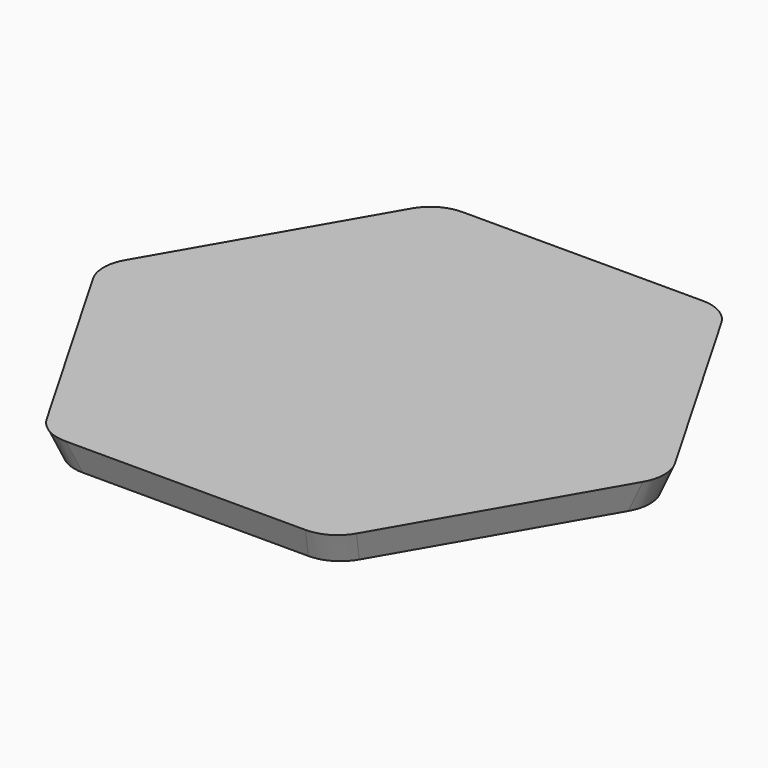
from build123d import *

# Parameters (mm, degrees)
F1_DEPTH = 5
F1_TAPER = -30
F3_DEPTH = 3
F3_TAPER = 30
F4_R     = 47.5
F5_DEPTH = 7
F5_TAPER = 22.5
F6_R     = 10


with BuildPart() as f1:
    # F0 (on Top) → F1 (new body)
    with BuildSketch(Plane.XY):
        Polygon((31.25, -54.1265877365), (62.5, 0), (31.25, 54.1265877365), (-31.25, 54.1265877365), (-62.5, 0), (-31.25, -54.1265877365), align=None)
    extrude(amount=F1_DEPTH, taper=F1_TAPER)

    # F2 (on face) → F3 (cut)
    with BuildSketch(Plane(origin=(0, 0, 0), x_dir=(1, 0, 0), z_dir=(0, 0, -1))):
        Polygon((61.1051684355, 65.1476408745), (58.6051684355, 60.8175138556), (61.1051684355, 56.4873868367), (66.1051684355, 56.4873868367), (68.6051684355, 60.8175138556), (66.1051684355, 65.1476408745), align=None)
        Polygon((51.440104926, 70.7277678934), (48.940104926, 66.3976408745), (51.440104926, 62.0675138556), (56.440104926, 62.0675138556), (58.940104926, 66.3976408745), (56.440104926, 70.7277678934), align=None)
        Polygon((48.940104926, 55.2376408745), (51.440104926, 50.9075138556), (56.440104926, 50.9075138556), (58.940104926, 55.2376408745), (56.440104926, 59.5677678934), (51.440104926, 59.5677678934), align=None)
        Polygon((66.1051684355, 53.9876408745), (61.1051684355, 53.9876408745), (58.6051684355, 49.6575138556), (61.1051684355, 45.3273868367), (66.1051684355, 45.3273868367), (68.6051684355, 49.6575138556), align=None)
        Polygon((48.940104926, 44.0776408745), (51.440104926, 39.7475138556), (56.440104926, 39.7475138556), (58.940104926, 44.0776408745), (56.440104926, 48.4077678934), (51.440104926, 48.4077678934), align=None)
        Polygon((66.1051684355, 42.8276408745), (61.1051684355, 42.8276408745), (58.6051684355, 38.4975138556), (61.1051684355, 34.1673868367), (66.1051684355, 34.1673868367), (68.6051684355, 38.4975138556), align=None)
        Polygon((48.940104926, 32.9176408745), (51.440104926, 28.5875138556), (56.440104926, 28.5875138556), (58.940104926, 32.9176408745), (56.440104926, 37.2477678934), (51.440104926, 37.2477678934), align=None)
        Polygon((66.1051684355, 31.6676408745), (61.1051684355, 31.6676408745), (58.6051684355, 27.3375138556), (61.1051684355, 23.0073868367), (66.1051684355, 23.0073868367), (68.6051684355, 27.3375138556), align=None)
        Polygon((48.940104926, 21.7576408745), (51.440104926, 17.4275138556), (56.440104926, 17.4275138556), (58.940104926, 21.7576408745), (56.440104926, 26.0877678934), (51.440104926, 26.0877678934), align=None)
        Polygon((66.1051684355, 20.5076408745), (61.1051684355, 20.5076408745), (58.6051684355, 16.1775138556), (61.1051684355, 11.8473868367), (66.1051684355, 11.8473868367), (68.6051684355, 16.1775138556), align=None)
        Polygon((48.940104926, 10.5976408745), (51.440104926, 6.2675138556), (56.440104926, 6.2675138556), (58.940104926, 10.5976408745), (56.440104926, 14.9277678934), (51.440104926, 14.9277678934), align=None)
        Polygon((66.1051684355, 9.3476408745), (61.1051684355, 9.3476408745), (58.6051684355, 5.0175138556), (61.1051684355, 0.6873868367), (66.1051684355, 0.6873868367), (68.6051684355, 5.0175138556), align=None)
        Polygon((48.940104926, -0.5623591255), (51.440104926, -4.8924861444), (56.440104926, -4.8924861444), (58.940104926, -0.5623591255), (56.440104926, 3.7677678934), (51.440104926, 3.7677678934), align=None)
        Polygon((66.1051684355, -1.8123591255), (61.1051684355, -1.8123591255), (58.6051684355, -6.1424861444), (61.1051684355, -10.4726131633), (66.1051684355, -10.4726131633), (68.6051684355, -6.1424861444), align=None)
        Polygon((48.940104926, -11.7223591255), (51.440104926, -16.0524861444), (56.440104926, -16.0524861444), (58.940104926, -11.7223591255), (56.440104926, -7.3922321066), (51.440104926, -7.3922321066), align=None)
        Polygon((66.1051684355, -12.9723591255), (61.1051684355, -12.9723591255), (58.6051684355, -17.3024861444), (61.1051684355, -21.6326131633), (66.1051684355, -21.6326131633), (68.6051684355, -17.3024861444), align=None)
        Polygon((48.940104926, -22.8823591255), (51.440104926, -27.2124861444), (56.440104926, -27.2124861444), (58.940104926, -22.8823591255), (56.440104926, -18.5522321066), (51.440104926, -18.5522321066), align=None)
        Polygon((66.1051684355, -24.1323591255), (61.1051684355, -24.1323591255), (58.6051684355, -28.4624861444), (61.1051684355, -32.7926131633), (66.1051684355, -32.7926131633), (68.6051684355, -28.4624861444), align=None)
        Polygon((48.940104926, -34.0423591255), (51.440104926, -38.3724861444), (56.440104926, -38.3724861444), (58.940104926, -34.0423591255), (56.440104926, -29.7122321066), (51.440104926, -29.7122321066), align=None)
        Polygon((66.1051684355, -35.2923591255), (61.1051684355, -35.2923591255), (58.6051684355, -39.6224861444), (61.1051684355, -43.9526131633), (66.1051684355, -43.9526131633), (68.6051684355, -39.6224861444), align=None)
        Polygon((48.940104926, -45.2023591255), (51.440104926, -49.5324861444), (56.440104926, -49.5324861444), (58.940104926, -45.2023591255), (56.440104926, -40.8722321066), (51.440104926, -40.8722321066), align=None)
        Polygon((66.1051684355, -46.4523591255), (61.1051684355, -46.4523591255), (58.6051684355, -50.7824861444), (61.1051684355, -55.1126131633), (66.1051684355, -55.1126131633), (68.6051684355, -50.7824861444), align=None)
        Polygon((28.940104926, 66.3976408745), (31.440104926, 62.0675138556), (36.440104926, 62.0675138556), (38.940104926, 66.3976408745), (36.440104926, 70.7277678934), (31.440104926, 70.7277678934), align=None)
        Polygon((46.1051684355, 65.1476408745), (41.1051684355, 65.1476408745), (38.6051684355, 60.8175138556), (41.1051684355, 56.4873868367), (46.1051684355, 56.4873868367), (48.6051684355, 60.8175138556), align=None)
        Polygon((28.940104926, 55.2376408745), (31.440104926, 50.9075138556), (36.440104926, 50.9075138556), (38.940104926, 55.2376408745), (36.440104926, 59.5677678934), (31.440104926, 59.5677678934), align=None)
        Polygon((46.1051684355, 53.9876408745), (41.1051684355, 53.9876408745), (38.6051684355, 49.6575138556), (41.1051684355, 45.3273868367), (46.1051684355, 45.3273868367), (48.6051684355, 49.6575138556), align=None)
        Polygon((28.940104926, 44.0776408745), (31.440104926, 39.7475138556), (36.440104926, 39.7475138556), (38.940104926, 44.0776408745), (36.440104926, 48.4077678934), (31.440104926, 48.4077678934), align=None)
        Polygon((46.1051684355, 42.8276408745), (41.1051684355, 42.8276408745), (38.6051684355, 38.4975138556), (41.1051684355, 34.1673868367), (46.1051684355, 34.1673868367), (48.6051684355, 38.4975138556), align=None)
        Polygon((28.940104926, 32.9176408745), (31.440104926, 28.5875138556), (36.440104926, 28.5875138556), (38.940104926, 32.9176408745), (36.440104926, 37.2477678934), (31.440104926, 37.2477678934), align=None)
        Polygon((46.1051684355, 31.6676408745), (41.1051684355, 31.6676408745), (38.6051684355, 27.3375138556), (41.1051684355, 23.0073868367), (46.1051684355, 23.0073868367), (48.6051684355, 27.3375138556), align=None)
        Polygon((28.940104926, 21.7576408745), (31.440104926, 17.4275138556), (36.440104926, 17.4275138556), (38.940104926, 21.7576408745), (36.440104926, 26.0877678934), (31.440104926, 26.0877678934), align=None)
        Polygon((46.1051684355, 20.5076408745), (41.1051684355, 20.5076408745), (38.6051684355, 16.1775138556), (41.1051684355, 11.8473868367), (46.1051684355, 11.8473868367), (48.6051684355, 16.1775138556), align=None)
        Polygon((28.940104926, 10.5976408745), (31.440104926, 6.2675138556), (36.440104926, 6.2675138556), (38.940104926, 10.5976408745), (36.440104926, 14.9277678934), (31.440104926, 14.9277678934), align=None)
        Polygon((46.1051684355, 9.3476408745), (41.1051684355, 9.3476408745), (38.6051684355, 5.0175138556), (41.1051684355, 0.6873868367), (46.1051684355, 0.6873868367), (48.6051684355, 5.0175138556), align=None)
        Polygon((28.940104926, -0.5623591255), (31.440104926, -4.8924861444), (36.440104926, -4.8924861444), (38.940104926, -0.5623591255), (36.440104926, 3.7677678934), (31.440104926, 3.7677678934), align=None)
        Polygon((46.1051684355, -1.8123591255), (41.1051684355, -1.8123591255), (38.6051684355, -6.1424861444), (41.1051684355, -10.4726131633), (46.1051684355, -10.4726131633), (48.6051684355, -6.1424861444), align=None)
        Polygon((28.940104926, -11.7223591255), (31.440104926, -16.0524861444), (36.440104926, -16.0524861444), (38.940104926, -11.7223591255), (36.440104926, -7.3922321066), (31.440104926, -7.3922321066), align=None)
        Polygon((46.1051684355, -12.9723591255), (41.1051684355, -12.9723591255), (38.6051684355, -17.3024861444), (41.1051684355, -21.6326131633), (46.1051684355, -21.6326131633), (48.6051684355, -17.3024861444), align=None)
        Polygon((28.940104926, -22.8823591255), (31.440104926, -27.2124861444), (36.440104926, -27.2124861444), (38.940104926, -22.8823591255), (36.440104926, -18.5522321066), (31.440104926, -18.5522321066), align=None)
        Polygon((46.1051684355, -24.1323591255), (41.1051684355, -24.1323591255), (38.6051684355, -28.4624861444), (41.1051684355, -32.7926131633), (46.1051684355, -32.7926131633), (48.6051684355, -28.4624861444), align=None)
        Polygon((28.940104926, -34.0423591255), (31.440104926, -38.3724861444), (36.440104926, -38.3724861444), (38.940104926, -34.0423591255), (36.440104926, -29.7122321066), (31.440104926, -29.7122321066), align=None)
        Polygon((46.1051684355, -35.2923591255), (41.1051684355, -35.2923591255), (38.6051684355, -39.6224861444), (41.1051684355, -43.9526131633), (46.1051684355, -43.9526131633), (48.6051684355, -39.6224861444), align=None)
        Polygon((28.940104926, -45.2023591255), (31.440104926, -49.5324861444), (36.440104926, -49.5324861444), (38.940104926, -45.2023591255), (36.440104926, -40.8722321066), (31.440104926, -40.8722321066), align=None)
        Polygon((46.1051684355, -46.4523591255), (41.1051684355, -46.4523591255), (38.6051684355, -50.7824861444), (41.1051684355, -55.1126131633), (46.1051684355, -55.1126131633), (48.6051684355, -50.7824861444), align=None)
        Polygon((8.940104926, 66.3976408745), (11.440104926, 62.0675138556), (16.440104926, 62.0675138556), (18.940104926, 66.3976408745), (16.440104926, 70.7277678934), (11.440104926, 70.7277678934), align=None)
        Polygon((26.1051684355, 65.1476408745), (21.1051684355, 65.1476408745), (18.6051684355, 60.8175138556), (21.1051684355, 56.4873868367), (26.1051684355, 56.4873868367), (28.6051684355, 60.8175138556), align=None)
        Polygon((8.940104926, 55.2376408745), (11.440104926, 50.9075138556), (16.440104926, 50.9075138556), (18.940104926, 55.2376408745), (16.440104926, 59.5677678934), (11.440104926, 59.5677678934), align=None)
        Polygon((26.1051684355, 53.9876408745), (21.1051684355, 53.9876408745), (18.6051684355, 49.6575138556), (21.1051684355, 45.3273868367), (26.1051684355, 45.3273868367), (28.6051684355, 49.6575138556), align=None)
        Polygon((8.940104926, 44.0776408745), (11.440104926, 39.7475138556), (16.440104926, 39.7475138556), (18.940104926, 44.0776408745), (16.440104926, 48.4077678934), (11.440104926, 48.4077678934), align=None)
        Polygon((26.1051684355, 42.8276408745), (21.1051684355, 42.8276408745), (18.6051684355, 38.4975138556), (21.1051684355, 34.1673868367), (26.1051684355, 34.1673868367), (28.6051684355, 38.4975138556), align=None)
        Polygon((8.940104926, 32.9176408745), (11.440104926, 28.5875138556), (16.440104926, 28.5875138556), (18.940104926, 32.9176408745), (16.440104926, 37.2477678934), (11.440104926, 37.2477678934), align=None)
        Polygon((26.1051684355, 31.6676408745), (21.1051684355, 31.6676408745), (18.6051684355, 27.3375138556), (21.1051684355, 23.0073868367), (26.1051684355, 23.0073868367), (28.6051684355, 27.3375138556), align=None)
        Polygon((8.940104926, 21.7576408745), (11.440104926, 17.4275138556), (16.440104926, 17.4275138556), (18.940104926, 21.7576408745), (16.440104926, 26.0877678934), (11.440104926, 26.0877678934), align=None)
        Polygon((26.1051684355, 20.5076408745), (21.1051684355, 20.5076408745), (18.6051684355, 16.1775138556), (21.1051684355, 11.8473868367), (26.1051684355, 11.8473868367), (28.6051684355, 16.1775138556), align=None)
        Polygon((8.940104926, 10.5976408745), (11.440104926, 6.2675138556), (16.440104926, 6.2675138556), (18.940104926, 10.5976408745), (16.440104926, 14.9277678934), (11.440104926, 14.9277678934), align=None)
        Polygon((26.1051684355, 9.3476408745), (21.1051684355, 9.3476408745), (18.6051684355, 5.0175138556), (21.1051684355, 0.6873868367), (26.1051684355, 0.6873868367), (28.6051684355, 5.0175138556), align=None)
        Polygon((8.940104926, -0.5623591255), (11.440104926, -4.8924861444), (16.440104926, -4.8924861444), (18.940104926, -0.5623591255), (16.440104926, 3.7677678934), (11.440104926, 3.7677678934), align=None)
        Polygon((26.1051684355, -1.8123591255), (21.1051684355, -1.8123591255), (18.6051684355, -6.1424861444), (21.1051684355, -10.4726131633), (26.1051684355, -10.4726131633), (28.6051684355, -6.1424861444), align=None)
        Polygon((8.940104926, -11.7223591255), (11.440104926, -16.0524861444), (16.440104926, -16.0524861444), (18.940104926, -11.7223591255), (16.440104926, -7.3922321066), (11.440104926, -7.3922321066), align=None)
        Polygon((26.1051684355, -12.9723591255), (21.1051684355, -12.9723591255), (18.6051684355, -17.3024861444), (21.1051684355, -21.6326131633), (26.1051684355, -21.6326131633), (28.6051684355, -17.3024861444), align=None)
        Polygon((8.940104926, -22.8823591255), (11.440104926, -27.2124861444), (16.440104926, -27.2124861444), (18.940104926, -22.8823591255), (16.440104926, -18.5522321066), (11.440104926, -18.5522321066), align=None)
        Polygon((26.1051684355, -24.1323591255), (21.1051684355, -24.1323591255), (18.6051684355, -28.4624861444), (21.1051684355, -32.7926131633), (26.1051684355, -32.7926131633), (28.6051684355, -28.4624861444), align=None)
        Polygon((8.940104926, -34.0423591255), (11.440104926, -38.3724861444), (16.440104926, -38.3724861444), (18.940104926, -34.0423591255), (16.440104926, -29.7122321066), (11.440104926, -29.7122321066), align=None)
        Polygon((26.1051684355, -35.2923591255), (21.1051684355, -35.2923591255), (18.6051684355, -39.6224861444), (21.1051684355, -43.9526131633), (26.1051684355, -43.9526131633), (28.6051684355, -39.6224861444), align=None)
        Polygon((8.940104926, -45.2023591255), (11.440104926, -49.5324861444), (16.440104926, -49.5324861444), (18.940104926, -45.2023591255), (16.440104926, -40.8722321066), (11.440104926, -40.8722321066), align=None)
        Polygon((26.1051684355, -46.4523591255), (21.1051684355, -46.4523591255), (18.6051684355, -50.7824861444), (21.1051684355, -55.1126131633), (26.1051684355, -55.1126131633), (28.6051684355, -50.7824861444), align=None)
        Polygon((-11.059895074, 66.3976408745), (-8.559895074, 62.0675138556), (-3.559895074, 62.0675138556), (-1.059895074, 66.3976408745), (-3.559895074, 70.7277678934), (-8.559895074, 70.7277678934), align=None)
        Polygon((6.1051684355, 65.1476408745), (1.1051684355, 65.1476408745), (-1.3948315645, 60.8175138556), (1.1051684355, 56.4873868367), (6.1051684355, 56.4873868367), (8.6051684355, 60.8175138556), align=None)
        Polygon((-11.059895074, 55.2376408745), (-8.559895074, 50.9075138556), (-3.559895074, 50.9075138556), (-1.059895074, 55.2376408745), (-3.559895074, 59.5677678934), (-8.559895074, 59.5677678934), align=None)
        Polygon((6.1051684355, 53.9876408745), (1.1051684355, 53.9876408745), (-1.3948315645, 49.6575138556), (1.1051684355, 45.3273868367), (6.1051684355, 45.3273868367), (8.6051684355, 49.6575138556), align=None)
        Polygon((-11.059895074, 44.0776408745), (-8.559895074, 39.7475138556), (-3.559895074, 39.7475138556), (-1.059895074, 44.0776408745), (-3.559895074, 48.4077678934), (-8.559895074, 48.4077678934), align=None)
        Polygon((6.1051684355, 42.8276408745), (1.1051684355, 42.8276408745), (-1.3948315645, 38.4975138556), (1.1051684355, 34.1673868367), (6.1051684355, 34.1673868367), (8.6051684355, 38.4975138556), align=None)
        Polygon((-11.059895074, 32.9176408745), (-8.559895074, 28.5875138556), (-3.559895074, 28.5875138556), (-1.059895074, 32.9176408745), (-3.559895074, 37.2477678934), (-8.559895074, 37.2477678934), align=None)
        Polygon((6.1051684355, 31.6676408745), (1.1051684355, 31.6676408745), (-1.3948315645, 27.3375138556), (1.1051684355, 23.0073868367), (6.1051684355, 23.0073868367), (8.6051684355, 27.3375138556), align=None)
        Polygon((-11.059895074, 21.7576408745), (-8.559895074, 17.4275138556), (-3.559895074, 17.4275138556), (-1.059895074, 21.7576408745), (-3.559895074, 26.0877678934), (-8.559895074, 26.0877678934), align=None)
        Polygon((6.1051684355, 20.5076408745), (1.1051684355, 20.5076408745), (-1.3948315645, 16.1775138556), (1.1051684355, 11.8473868367), (6.1051684355, 11.8473868367), (8.6051684355, 16.1775138556), align=None)
        Polygon((-11.059895074, 10.5976408745), (-8.559895074, 6.2675138556), (-3.559895074, 6.2675138556), (-1.059895074, 10.5976408745), (-3.559895074, 14.9277678934), (-8.559895074, 14.9277678934), align=None)
        Polygon((6.1051684355, 9.3476408745), (1.1051684355, 9.3476408745), (-1.3948315645, 5.0175138556), (1.1051684355, 0.6873868367), (6.1051684355, 0.6873868367), (8.6051684355, 5.0175138556), align=None)
        Polygon((-11.059895074, -0.5623591255), (-8.559895074, -4.8924861444), (-3.559895074, -4.8924861444), (-1.059895074, -0.5623591255), (-3.559895074, 3.7677678934), (-8.559895074, 3.7677678934), align=None)
        Polygon((6.1051684355, -1.8123591255), (1.1051684355, -1.8123591255), (-1.3948315645, -6.1424861444), (1.1051684355, -10.4726131633), (6.1051684355, -10.4726131633), (8.6051684355, -6.1424861444), align=None)
        Polygon((-11.059895074, -11.7223591255), (-8.559895074, -16.0524861444), (-3.559895074, -16.0524861444), (-1.059895074, -11.7223591255), (-3.559895074, -7.3922321066), (-8.559895074, -7.3922321066), align=None)
        Polygon((6.1051684355, -12.9723591255), (1.1051684355, -12.9723591255), (-1.3948315645, -17.3024861444), (1.1051684355, -21.6326131633), (6.1051684355, -21.6326131633), (8.6051684355, -17.3024861444), align=None)
        Polygon((-11.059895074, -22.8823591255), (-8.559895074, -27.2124861444), (-3.559895074, -27.2124861444), (-1.059895074, -22.8823591255), (-3.559895074, -18.5522321066), (-8.559895074, -18.5522321066), align=None)
        Polygon((6.1051684355, -24.1323591255), (1.1051684355, -24.1323591255), (-1.3948315645, -28.4624861444), (1.1051684355, -32.7926131633), (6.1051684355, -32.7926131633), (8.6051684355, -28.4624861444), align=None)
        Polygon((-11.059895074, -34.0423591255), (-8.559895074, -38.3724861444), (-3.559895074, -38.3724861444), (-1.059895074, -34.0423591255), (-3.559895074, -29.7122321066), (-8.559895074, -29.7122321066), align=None)
        Polygon((6.1051684355, -35.2923591255), (1.1051684355, -35.2923591255), (-1.3948315645, -39.6224861444), (1.1051684355, -43.9526131633), (6.1051684355, -43.9526131633), (8.6051684355, -39.6224861444), align=None)
        Polygon((-11.059895074, -45.2023591255), (-8.559895074, -49.5324861444), (-3.559895074, -49.5324861444), (-1.059895074, -45.2023591255), (-3.559895074, -40.8722321066), (-8.559895074, -40.8722321066), align=None)
        Polygon((6.1051684355, -46.4523591255), (1.1051684355, -46.4523591255), (-1.3948315645, -50.7824861444), (1.1051684355, -55.1126131633), (6.1051684355, -55.1126131633), (8.6051684355, -50.7824861444), align=None)
        Polygon((-31.059895074, 66.3976408745), (-28.559895074, 62.0675138556), (-23.559895074, 62.0675138556), (-21.059895074, 66.3976408745), (-23.559895074, 70.7277678934), (-28.559895074, 70.7277678934), align=None)
        Polygon((-13.8948315645, 65.1476408745), (-18.8948315645, 65.1476408745), (-21.3948315645, 60.8175138556), (-18.8948315645, 56.4873868367), (-13.8948315645, 56.4873868367), (-11.3948315645, 60.8175138556), align=None)
        Polygon((-31.059895074, 55.2376408745), (-28.559895074, 50.9075138556), (-23.559895074, 50.9075138556), (-21.059895074, 55.2376408745), (-23.559895074, 59.5677678934), (-28.559895074, 59.5677678934), align=None)
        Polygon((-13.8948315645, 53.9876408745), (-18.8948315645, 53.9876408745), (-21.3948315645, 49.6575138556), (-18.8948315645, 45.3273868367), (-13.8948315645, 45.3273868367), (-11.3948315645, 49.6575138556), align=None)
        Polygon((-31.059895074, 44.0776408745), (-28.559895074, 39.7475138556), (-23.559895074, 39.7475138556), (-21.059895074, 44.0776408745), (-23.559895074, 48.4077678934), (-28.559895074, 48.4077678934), align=None)
        Polygon((-13.8948315645, 42.8276408745), (-18.8948315645, 42.8276408745), (-21.3948315645, 38.4975138556), (-18.8948315645, 34.1673868367), (-13.8948315645, 34.1673868367), (-11.3948315645, 38.4975138556), align=None)
        Polygon((-31.059895074, 32.9176408745), (-28.559895074, 28.5875138556), (-23.559895074, 28.5875138556), (-21.059895074, 32.9176408745), (-23.559895074, 37.2477678934), (-28.559895074, 37.2477678934), align=None)
        Polygon((-13.8948315645, 31.6676408745), (-18.8948315645, 31.6676408745), (-21.3948315645, 27.3375138556), (-18.8948315645, 23.0073868367), (-13.8948315645, 23.0073868367), (-11.3948315645, 27.3375138556), align=None)
        Polygon((-31.059895074, 21.7576408745), (-28.559895074, 17.4275138556), (-23.559895074, 17.4275138556), (-21.059895074, 21.7576408745), (-23.559895074, 26.0877678934), (-28.559895074, 26.0877678934), align=None)
        Polygon((-13.8948315645, 20.5076408745), (-18.8948315645, 20.5076408745), (-21.3948315645, 16.1775138556), (-18.8948315645, 11.8473868367), (-13.8948315645, 11.8473868367), (-11.3948315645, 16.1775138556), align=None)
        Polygon((-31.059895074, 10.5976408745), (-28.559895074, 6.2675138556), (-23.559895074, 6.2675138556), (-21.059895074, 10.5976408745), (-23.559895074, 14.9277678934), (-28.559895074, 14.9277678934), align=None)
        Polygon((-13.8948315645, 9.3476408745), (-18.8948315645, 9.3476408745), (-21.3948315645, 5.0175138556), (-18.8948315645, 0.6873868367), (-13.8948315645, 0.6873868367), (-11.3948315645, 5.0175138556), align=None)
        Polygon((-31.059895074, -0.5623591255), (-28.559895074, -4.8924861444), (-23.559895074, -4.8924861444), (-21.059895074, -0.5623591255), (-23.559895074, 3.7677678934), (-28.559895074, 3.7677678934), align=None)
        Polygon((-13.8948315645, -1.8123591255), (-18.8948315645, -1.8123591255), (-21.3948315645, -6.1424861444), (-18.8948315645, -10.4726131633), (-13.8948315645, -10.4726131633), (-11.3948315645, -6.1424861444), align=None)
        Polygon((-31.059895074, -11.7223591255), (-28.559895074, -16.0524861444), (-23.559895074, -16.0524861444), (-21.059895074, -11.7223591255), (-23.559895074, -7.3922321066), (-28.559895074, -7.3922321066), align=None)
        Polygon((-13.8948315645, -12.9723591255), (-18.8948315645, -12.9723591255), (-21.3948315645, -17.3024861444), (-18.8948315645, -21.6326131633), (-13.8948315645, -21.6326131633), (-11.3948315645, -17.3024861444), align=None)
        Polygon((-31.059895074, -22.8823591255), (-28.559895074, -27.2124861444), (-23.559895074, -27.2124861444), (-21.059895074, -22.8823591255), (-23.559895074, -18.5522321066), (-28.559895074, -18.5522321066), align=None)
        Polygon((-13.8948315645, -24.1323591255), (-18.8948315645, -24.1323591255), (-21.3948315645, -28.4624861444), (-18.8948315645, -32.7926131633), (-13.8948315645, -32.7926131633), (-11.3948315645, -28.4624861444), align=None)
        Polygon((-31.059895074, -34.0423591255), (-28.559895074, -38.3724861444), (-23.559895074, -38.3724861444), (-21.059895074, -34.0423591255), (-23.559895074, -29.7122321066), (-28.559895074, -29.7122321066), align=None)
        Polygon((-13.8948315645, -35.2923591255), (-18.8948315645, -35.2923591255), (-21.3948315645, -39.6224861444), (-18.8948315645, -43.9526131633), (-13.8948315645, -43.9526131633), (-11.3948315645, -39.6224861444), align=None)
        Polygon((-31.059895074, -45.2023591255), (-28.559895074, -49.5324861444), (-23.559895074, -49.5324861444), (-21.059895074, -45.2023591255), (-23.559895074, -40.8722321066), (-28.559895074, -40.8722321066), align=None)
        Polygon((-13.8948315645, -46.4523591255), (-18.8948315645, -46.4523591255), (-21.3948315645, -50.7824861444), (-18.8948315645, -55.1126131633), (-13.8948315645, -55.1126131633), (-11.3948315645, -50.7824861444), align=None)
        Polygon((-51.059895074, 66.3976408745), (-48.559895074, 62.0675138556), (-43.559895074, 62.0675138556), (-41.059895074, 66.3976408745), (-43.559895074, 70.7277678934), (-48.559895074, 70.7277678934), align=None)
        Polygon((-33.8948315645, 65.1476408745), (-38.8948315645, 65.1476408745), (-41.3948315645, 60.8175138556), (-38.8948315645, 56.4873868367), (-33.8948315645, 56.4873868367), (-31.3948315645, 60.8175138556), align=None)
        Polygon((-51.059895074, 55.2376408745), (-48.559895074, 50.9075138556), (-43.559895074, 50.9075138556), (-41.059895074, 55.2376408745), (-43.559895074, 59.5677678934), (-48.559895074, 59.5677678934), align=None)
        Polygon((-33.8948315645, 53.9876408745), (-38.8948315645, 53.9876408745), (-41.3948315645, 49.6575138556), (-38.8948315645, 45.3273868367), (-33.8948315645, 45.3273868367), (-31.3948315645, 49.6575138556), align=None)
        Polygon((-51.059895074, 44.0776408745), (-48.559895074, 39.7475138556), (-43.559895074, 39.7475138556), (-41.059895074, 44.0776408745), (-43.559895074, 48.4077678934), (-48.559895074, 48.4077678934), align=None)
        Polygon((-33.8948315645, 42.8276408745), (-38.8948315645, 42.8276408745), (-41.3948315645, 38.4975138556), (-38.8948315645, 34.1673868367), (-33.8948315645, 34.1673868367), (-31.3948315645, 38.4975138556), align=None)
        Polygon((-51.059895074, 32.9176408745), (-48.559895074, 28.5875138556), (-43.559895074, 28.5875138556), (-41.059895074, 32.9176408745), (-43.559895074, 37.2477678934), (-48.559895074, 37.2477678934), align=None)
        Polygon((-33.8948315645, 31.6676408745), (-38.8948315645, 31.6676408745), (-41.3948315645, 27.3375138556), (-38.8948315645, 23.0073868367), (-33.8948315645, 23.0073868367), (-31.3948315645, 27.3375138556), align=None)
        Polygon((-51.059895074, 21.7576408745), (-48.559895074, 17.4275138556), (-43.559895074, 17.4275138556), (-41.059895074, 21.7576408745), (-43.559895074, 26.0877678934), (-48.559895074, 26.0877678934), align=None)
        Polygon((-33.8948315645, 20.5076408745), (-38.8948315645, 20.5076408745), (-41.3948315645, 16.1775138556), (-38.8948315645, 11.8473868367), (-33.8948315645, 11.8473868367), (-31.3948315645, 16.1775138556), align=None)
        Polygon((-51.059895074, 10.5976408745), (-48.559895074, 6.2675138556), (-43.559895074, 6.2675138556), (-41.059895074, 10.5976408745), (-43.559895074, 14.9277678934), (-48.559895074, 14.9277678934), align=None)
        Polygon((-33.8948315645, 9.3476408745), (-38.8948315645, 9.3476408745), (-41.3948315645, 5.0175138556), (-38.8948315645, 0.6873868367), (-33.8948315645, 0.6873868367), (-31.3948315645, 5.0175138556), align=None)
        Polygon((-51.059895074, -0.5623591255), (-48.559895074, -4.8924861444), (-43.559895074, -4.8924861444), (-41.059895074, -0.5623591255), (-43.559895074, 3.7677678934), (-48.559895074, 3.7677678934), align=None)
        Polygon((-33.8948315645, -1.8123591255), (-38.8948315645, -1.8123591255), (-41.3948315645, -6.1424861444), (-38.8948315645, -10.4726131633), (-33.8948315645, -10.4726131633), (-31.3948315645, -6.1424861444), align=None)
        Polygon((-51.059895074, -11.7223591255), (-48.559895074, -16.0524861444), (-43.559895074, -16.0524861444), (-41.059895074, -11.7223591255), (-43.559895074, -7.3922321066), (-48.559895074, -7.3922321066), align=None)
        Polygon((-33.8948315645, -12.9723591255), (-38.8948315645, -12.9723591255), (-41.3948315645, -17.3024861444), (-38.8948315645, -21.6326131633), (-33.8948315645, -21.6326131633), (-31.3948315645, -17.3024861444), align=None)
        Polygon((-51.059895074, -22.8823591255), (-48.559895074, -27.2124861444), (-43.559895074, -27.2124861444), (-41.059895074, -22.8823591255), (-43.559895074, -18.5522321066), (-48.559895074, -18.5522321066), align=None)
        Polygon((-33.8948315645, -24.1323591255), (-38.8948315645, -24.1323591255), (-41.3948315645, -28.4624861444), (-38.8948315645, -32.7926131633), (-33.8948315645, -32.7926131633), (-31.3948315645, -28.4624861444), align=None)
        Polygon((-51.059895074, -34.0423591255), (-48.559895074, -38.3724861444), (-43.559895074, -38.3724861444), (-41.059895074, -34.0423591255), (-43.559895074, -29.7122321066), (-48.559895074, -29.7122321066), align=None)
        Polygon((-33.8948315645, -35.2923591255), (-38.8948315645, -35.2923591255), (-41.3948315645, -39.6224861444), (-38.8948315645, -43.9526131633), (-33.8948315645, -43.9526131633), (-31.3948315645, -39.6224861444), align=None)
        Polygon((-51.059895074, -45.2023591255), (-48.559895074, -49.5324861444), (-43.559895074, -49.5324861444), (-41.059895074, -45.2023591255), (-43.559895074, -40.8722321066), (-48.559895074, -40.8722321066), align=None)
        Polygon((-33.8948315645, -46.4523591255), (-38.8948315645, -46.4523591255), (-41.3948315645, -50.7824861444), (-38.8948315645, -55.1126131633), (-33.8948315645, -55.1126131633), (-31.3948315645, -50.7824861444), align=None)
        Polygon((-71.059895074, 66.3976408745), (-68.559895074, 62.0675138556), (-63.559895074, 62.0675138556), (-61.059895074, 66.3976408745), (-63.559895074, 70.7277678934), (-68.559895074, 70.7277678934), align=None)
        Polygon((-53.8948315645, 65.1476408745), (-58.8948315645, 65.1476408745), (-61.3948315645, 60.8175138556), (-58.8948315645, 56.4873868367), (-53.8948315645, 56.4873868367), (-51.3948315645, 60.8175138556), align=None)
        Polygon((-71.059895074, 55.2376408745), (-68.559895074, 50.9075138556), (-63.559895074, 50.9075138556), (-61.059895074, 55.2376408745), (-63.559895074, 59.5677678934), (-68.559895074, 59.5677678934), align=None)
        Polygon((-53.8948315645, 53.9876408745), (-58.8948315645, 53.9876408745), (-61.3948315645, 49.6575138556), (-58.8948315645, 45.3273868367), (-53.8948315645, 45.3273868367), (-51.3948315645, 49.6575138556), align=None)
        Polygon((-71.059895074, 44.0776408745), (-68.559895074, 39.7475138556), (-63.559895074, 39.7475138556), (-61.059895074, 44.0776408745), (-63.559895074, 48.4077678934), (-68.559895074, 48.4077678934), align=None)
        Polygon((-53.8948315645, 42.8276408745), (-58.8948315645, 42.8276408745), (-61.3948315645, 38.4975138556), (-58.8948315645, 34.1673868367), (-53.8948315645, 34.1673868367), (-51.3948315645, 38.4975138556), align=None)
        Polygon((-71.059895074, 32.9176408745), (-68.559895074, 28.5875138556), (-63.559895074, 28.5875138556), (-61.059895074, 32.9176408745), (-63.559895074, 37.2477678934), (-68.559895074, 37.2477678934), align=None)
        Polygon((-53.8948315645, 31.6676408745), (-58.8948315645, 31.6676408745), (-61.3948315645, 27.3375138556), (-58.8948315645, 23.0073868367), (-53.8948315645, 23.0073868367), (-51.3948315645, 27.3375138556), align=None)
        Polygon((-71.059895074, 21.7576408745), (-68.559895074, 17.4275138556), (-63.559895074, 17.4275138556), (-61.059895074, 21.7576408745), (-63.559895074, 26.0877678934), (-68.559895074, 26.0877678934), align=None)
        Polygon((-53.8948315645, 20.5076408745), (-58.8948315645, 20.5076408745), (-61.3948315645, 16.1775138556), (-58.8948315645, 11.8473868367), (-53.8948315645, 11.8473868367), (-51.3948315645, 16.1775138556), align=None)
        Polygon((-71.059895074, 10.5976408745), (-68.559895074, 6.2675138556), (-63.559895074, 6.2675138556), (-61.059895074, 10.5976408745), (-63.559895074, 14.9277678934), (-68.559895074, 14.9277678934), align=None)
        Polygon((-53.8948315645, 9.3476408745), (-58.8948315645, 9.3476408745), (-61.3948315645, 5.0175138556), (-58.8948315645, 0.6873868367), (-53.8948315645, 0.6873868367), (-51.3948315645, 5.0175138556), align=None)
        Polygon((-71.059895074, -0.5623591255), (-68.559895074, -4.8924861444), (-63.559895074, -4.8924861444), (-61.059895074, -0.5623591255), (-63.559895074, 3.7677678934), (-68.559895074, 3.7677678934), align=None)
        Polygon((-53.8948315645, -1.8123591255), (-58.8948315645, -1.8123591255), (-61.3948315645, -6.1424861444), (-58.8948315645, -10.4726131633), (-53.8948315645, -10.4726131633), (-51.3948315645, -6.1424861444), align=None)
        Polygon((-71.059895074, -11.7223591255), (-68.559895074, -16.0524861444), (-63.559895074, -16.0524861444), (-61.059895074, -11.7223591255), (-63.559895074, -7.3922321066), (-68.559895074, -7.3922321066), align=None)
        Polygon((-53.8948315645, -12.9723591255), (-58.8948315645, -12.9723591255), (-61.3948315645, -17.3024861444), (-58.8948315645, -21.6326131633), (-53.8948315645, -21.6326131633), (-51.3948315645, -17.3024861444), align=None)
        Polygon((-71.059895074, -22.8823591255), (-68.559895074, -27.2124861444), (-63.559895074, -27.2124861444), (-61.059895074, -22.8823591255), (-63.559895074, -18.5522321066), (-68.559895074, -18.5522321066), align=None)
        Polygon((-53.8948315645, -24.1323591255), (-58.8948315645, -24.1323591255), (-61.3948315645, -28.4624861444), (-58.8948315645, -32.7926131633), (-53.8948315645, -32.7926131633), (-51.3948315645, -28.4624861444), align=None)
        Polygon((-71.059895074, -34.0423591255), (-68.559895074, -38.3724861444), (-63.559895074, -38.3724861444), (-61.059895074, -34.0423591255), (-63.559895074, -29.7122321066), (-68.559895074, -29.7122321066), align=None)
        Polygon((-53.8948315645, -35.2923591255), (-58.8948315645, -35.2923591255), (-61.3948315645, -39.6224861444), (-58.8948315645, -43.9526131633), (-53.8948315645, -43.9526131633), (-51.3948315645, -39.6224861444), align=None)
        Polygon((-71.059895074, -45.2023591255), (-68.559895074, -49.5324861444), (-63.559895074, -49.5324861444), (-61.059895074, -45.2023591255), (-63.559895074, -40.8722321066), (-68.559895074, -40.8722321066), align=None)
        Polygon((-53.8948315645, -46.4523591255), (-58.8948315645, -46.4523591255), (-61.3948315645, -50.7824861444), (-58.8948315645, -55.1126131633), (-53.8948315645, -55.1126131633), (-51.3948315645, -50.7824861444), align=None)
    extrude(amount=-F3_DEPTH, taper=F3_TAPER, mode=Mode.SUBTRACT)

    # F4 (on face) → F5 (join)
    with BuildSketch(Plane.XY.offset(5)):
        Polygon((32.9166666667, -57.0133390825), (65.8333333333, 0), (32.9166666667, 57.0133390825), (-32.9166666667, 57.0133390825), (-65.8333333333, 0), (-32.9166666667, -57.0133390825), align=None)
        Circle(F4_R, mode=Mode.SUBTRACT)
    extrude(amount=-F5_DEPTH, taper=F5_TAPER)

    # F6
    f6_edges = [f1.edges().sort_by_distance(p)[0] for p in [
        (32.079655, -55.563592, 1.5),
        (-32.079655, -55.563592, 1.5),
        (-64.159309, 0, 1.5),
        (64.159309, 0, 1.5),
        (-32.079655, 55.563592, 1.5),
        (32.079655, 55.563592, 1.5),
    ]]
    fillet(f6_edges, radius=F6_R)


solid = f1.part
